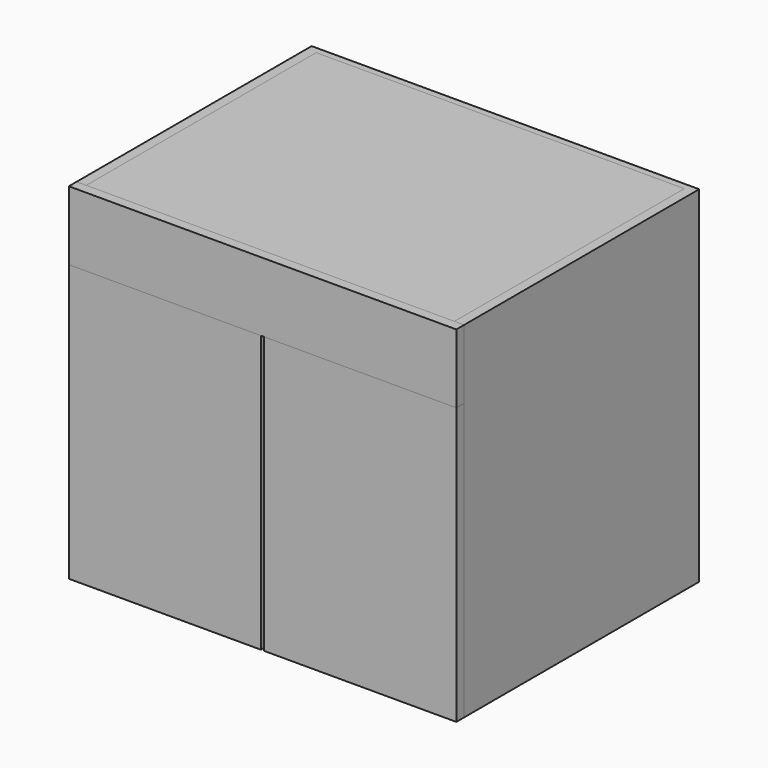
from build123d import *

# Parameters (mm, degrees)
F4_W      = 19.05
F4_H      = 565.15
F5_DEPTH  = 679.45
F6_W      = 723.9
F6_H      = 565.15
F7_DEPTH  = 19.05
F8_W      = 723.9
F8_H      = 565.15
F9_DEPTH  = 19.05
F10_W     = 762
F10_H     = 135.73125
F11_DEPTH = 19.05
F12_W     = 723.9
F12_H     = 19.05
F13_DEPTH = 565.15
F15_DEPTH = 19.05
F19_W     = 377.825
F19_H     = 543.71875
F20_DEPTH = 19.05


# Not quite as in the source:
# - a variable given as a bare number and used for a length is read in inches; the dataset says mm whatever the document's units were


with BuildPart() as f5:
    # F4 (on Top) → F5 (new body)
    with BuildSketch(Plane.XY):
        Polygon((762, 577.85), (0, 577.85), (0, 565.15), (19.05, 565.15), (742.95, 565.15), (762, 565.15), align=None)
        with Locations((9.525, 282.575)):
            Rectangle(F4_W, F4_H)
        with Locations((752.475, 282.575)):
            Rectangle(F4_W, F4_H)
    extrude(amount=-F5_DEPTH)


with BuildPart() as f7:
    # F6 (on Top) → F7 (new body)
    with BuildSketch(Plane.XY):
        with Locations((381, 282.575)):
            Rectangle(F6_W, F6_H)
    extrude(amount=-F7_DEPTH)


with BuildPart() as f9:
    # F8 (on face) → F9 (new body)
    with BuildSketch(Plane(origin=(0, 0, -679.45), x_dir=(1, 0, 0), z_dir=(0, 0, -1))):
        with Locations((381, -282.575)):
            Rectangle(F8_W, F8_H)
    extrude(amount=-F9_DEPTH)


with BuildPart() as f11:
    # F10 (on face) → F11 (new body)
    with BuildSketch(Plane.XZ):
        with Locations((381, -67.865625)):
            Rectangle(F10_W, F10_H)
    extrude(amount=F11_DEPTH)


with BuildPart() as f13:
    # F12 (on face) → F13 (new body)
    with BuildSketch(Plane.XZ.offset(-565.15)):
        with Locations((381, -349.25)):
            Rectangle(F12_W, F12_H)
    extrude(amount=F13_DEPTH)


with BuildPart() as f15:
    # F14 (on face) → F15 (new body)
    with BuildSketch(Plane.XZ):
        Polygon((762, -135.73125), (742.95, -135.73125), (742.95, -339.725), (742.95, -358.775), (742.95, -660.4), (742.95, -679.45), (762, -679.45), align=None)
        Polygon((742.95, -358.775), (742.95, -339.725), (19.05, -339.725), (19.05, -135.73125), (0, -135.73125), (0, -679.45), (19.05, -679.45), (742.95, -679.45), (742.95, -660.4), (19.05, -660.4), (19.05, -358.775), align=None)
    extrude(amount=F15_DEPTH)


with BuildPart() as f20:
    # F19 (on Front) → F20 (new body)
    with BuildSketch(Plane.XZ):
        with Locations((188.9125, -407.590625)):
            Rectangle(F19_W, F19_H)
    extrude(amount=F20_DEPTH)


with BuildPart() as f20b:
    # F19 (on Front) → F20, piece 2 (new body)
    with BuildSketch(Plane.XZ):
        with Locations((573.0875, -407.590625)):
            Rectangle(F19_W, F19_H)
    extrude(amount=F20_DEPTH)


solid = Compound([f5.part, f7.part, f9.part, f11.part, f20.part, f20b.part])
